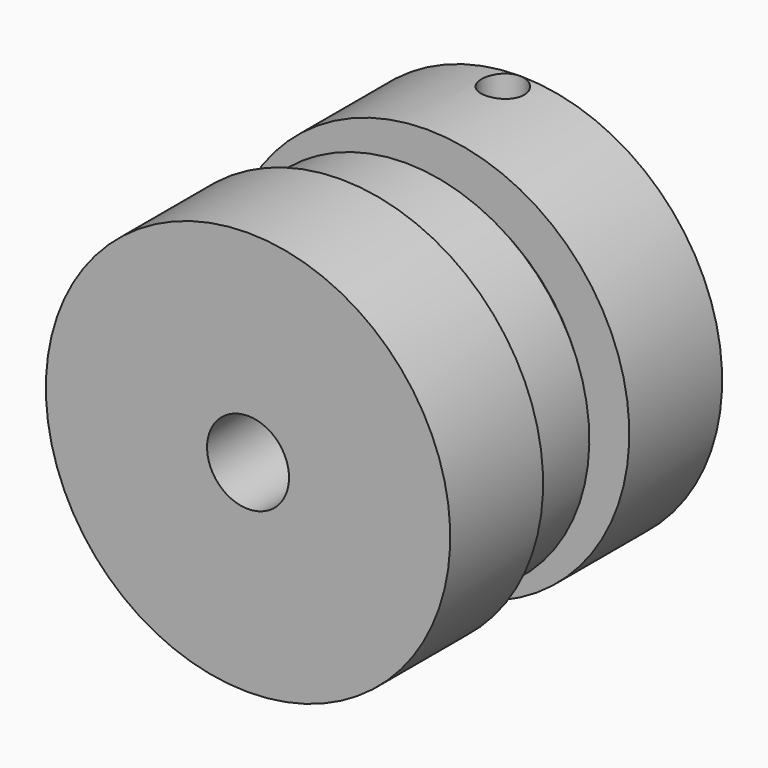
from build123d import *

# Parameters (mm, degrees)
F2_SIZE        = 3.175
F3_R           = 0.254
F6_D           = 5.1054
F6_DEPTH       = 49.3522
F6_START       = 0.2754562
F6_CBORE_D     = 10.414
F6_CBORE_DEPTH = 33.4772
F6_TIP         = 1.5338169022


# Not quite as in the source:
# - a feature names something its author has since deleted; it is built from what else it names


with BuildPart() as f1:
    # F0 (on Right) → F1 (revolve)
    with BuildSketch(Plane.YZ):
        Polygon((-41.4782, 10.0076), (0, 10.0076), (41.4782, 10.0076), (41.4782, 49.3522), (13.1445, 49.3522), (13.1445, 23.5712), (9.7155, 23.5712), (9.7155, 44.8818), (-13.1445, 44.8818), (-13.1445, 49.3522), (-41.4782, 49.3522), align=None)
    revolve(axis=Axis((0, -0.9843776588, 0), (0, 1, 0)))

    # F2
    f2_edges = [f1.edges().sort_by_distance(p)[0] for p in [
        (0, 9.7155, -44.8818),
    ]]
    chamfer(f2_edges, length=F2_SIZE)

    # F3
    f3_edges = [f1.edges().sort_by_distance(p)[0] for p in [
        (0, 9.7155, -23.5712),
        (0, 13.1445, -23.5712),
    ]]
    fillet(f3_edges, radius=F3_R)

    # F6
    # its depths count from where the whole tool has entered the part; down to there all is cleared
    with Locations(Plane.XY.offset(49.3522).offset(-F6_START)):
        with Locations((0, 36.2458)):
            CounterBoreHole(F6_D / 2, F6_CBORE_D / 2, F6_CBORE_DEPTH, depth=F6_DEPTH)
            with Locations((0, 0, -(F6_DEPTH + F6_TIP / 2))):  # 118° drill point
                Cone(0, F6_D / 2, F6_TIP, mode=Mode.SUBTRACT)


solid = f1.part
